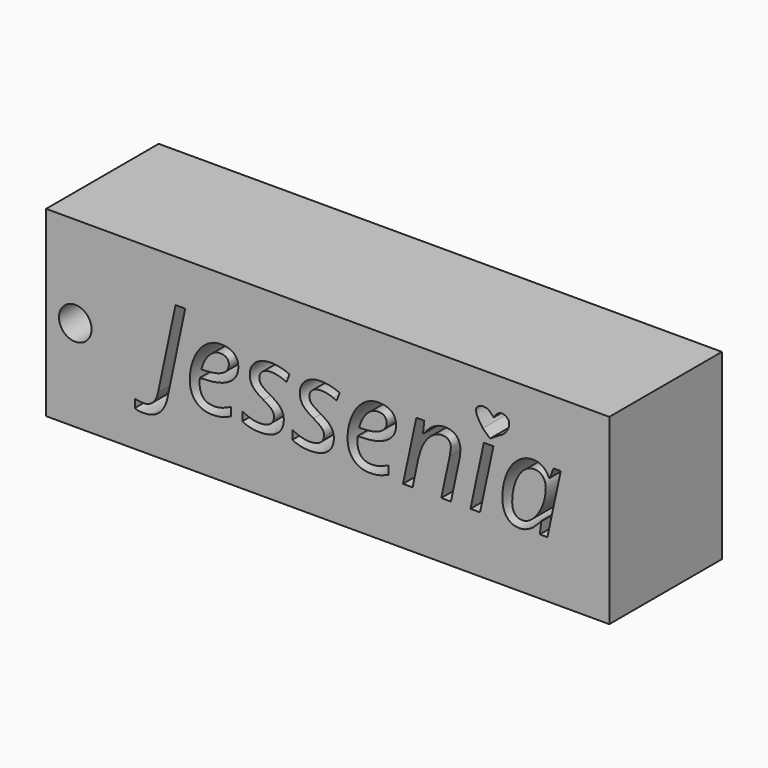
from build123d import *

# Parameters (mm, degrees)
F0_W         = 101.6
F0_H         = 32.9306531651
F2_DEPTH     = 25.4
F1_TEXT_SIZE = 21.0894161784
F3_DEPTH     = 25.4
F6_DEPTH     = 25.4
F7_R         = 2.9382667166
F8_DEPTH     = 25.4


# Not quite as in the source:
# - Text() gives the source's letters only with a copy of the font that has no kerning and outlines rounded to 1/6400 em; it was checked with that copy


with BuildPart() as f2:
    # F0 (on Front) → F2 (new body)
    with BuildSketch(Plane.XZ):
        with Locations((2.1698502951, 0)):
            Rectangle(F0_W, F0_H)
    extrude(amount=F2_DEPTH)

    # F1 (on face) → F3 (cut)
    with BuildSketch(Plane.XZ):
        with Locations((-29.3467342854, -6.2781567685)):
            Text('Jessenia', F1_TEXT_SIZE, font='Open Sans', font_style=FontStyle.ITALIC, text_align=(TextAlign.LEFT, TextAlign.BOTTOM))
    extrude(amount=F3_DEPTH, mode=Mode.SUBTRACT)

    # F5 (on face) → F6 (cut)
    with BuildSketch(Plane.XZ.offset(25.4)):
        with BuildLine():
            add(Edge.make_bspline(
                [(32.1269502951, 9.5880686721), (32.4671035601, 10.0416511055), (33.101917332, 11.1265729046), (35.7569755168, 10.0138094431), (34.2661740115, 7.5515914295), (33.3913937211, 7.2235497646)],
                knots=[0, 0, 0, 0, 0.2929993544, 0.6026795566, 1, 1, 1, 1], degree=3))
            add(Edge.make_bspline(
                [(32.1269502951, 9.5880686721), (31.7276213026, 10.0252756454), (30.9094892967, 11.0784480479), (28.1562248087, 10.2899544283), (29.3922569507, 8.3131357154), (30.1549676806, 7.2235497646)],
                knots=[0, 0, 0, 0, 0.302842276, 0.6040634249, 1, 1, 1, 1], degree=3))
            Line((30.1549676806, 7.2235497646), (31.4591015255, 6.0192301235))
            Line((31.4591015255, 6.0192301235), (33.3913937211, 7.2235497646))
        make_face()
    extrude(amount=-F6_DEPTH, mode=Mode.SUBTRACT)

    # F7 (on face) → F8 (cut)
    with BuildSketch(Plane.XZ.offset(25.4)):
        with Locations((-43.363083154, 0)):
            Circle(F7_R)
    extrude(amount=-F8_DEPTH, mode=Mode.SUBTRACT)


solid = f2.part
